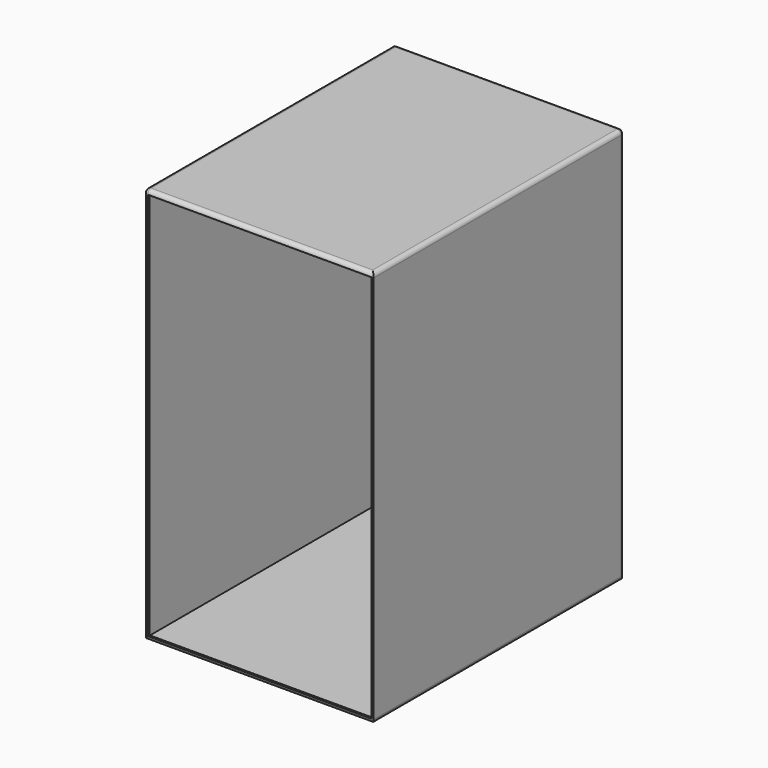
from build123d import *

# Parameters (mm, degrees)
F0_W     = 279.4
F0_H     = 482.6
F1_DEPTH = 381
F2_R     = 5
F3_T     = -2.54


# Not quite as in the source:
# - a shell that OpenCascade refuses in one call is made with other operations: the cavity is built on its own and cut out


with BuildPart() as f1:
    # F0 (on Front) → F1 (new body)
    with BuildSketch(Plane.XZ):
        Rectangle(F0_W, F0_H)
    extrude(amount=F1_DEPTH)

    # F2
    f2_edges = [f1.edges().sort_by_distance(p)[0] for p in [
        (139.7, -190.5, 241.3),
        (-139.7, -190.5, 241.3),
        (139.7, -190.5, -241.3),
        (139.7, 0, 0),
        (0, 0, 241.3),
        (-139.7, -381, 0),
        (0, -381, -241.3),
        (0, -381, 241.3),
    ]]
    fillet(f2_edges, radius=F2_R)

    # F3: a shell. OpenCascade refuses it in one call, so the cavity is built on its own and cut out:
    # the body offset inwards by the wall thickness, plus a prism from it out through each open face.
    f3_core = offset(f1.part, amount=F3_T, mode=Mode.PRIVATE)
    f3_exits = [f3_core.faces().sort_by_distance(p)[0] for p in [
        (1.23, -378.46, 0),
    ]]
    add(f3_core, mode=Mode.SUBTRACT)
    extrude(f3_exits, amount=-F3_T, mode=Mode.SUBTRACT)


solid = f1.part
